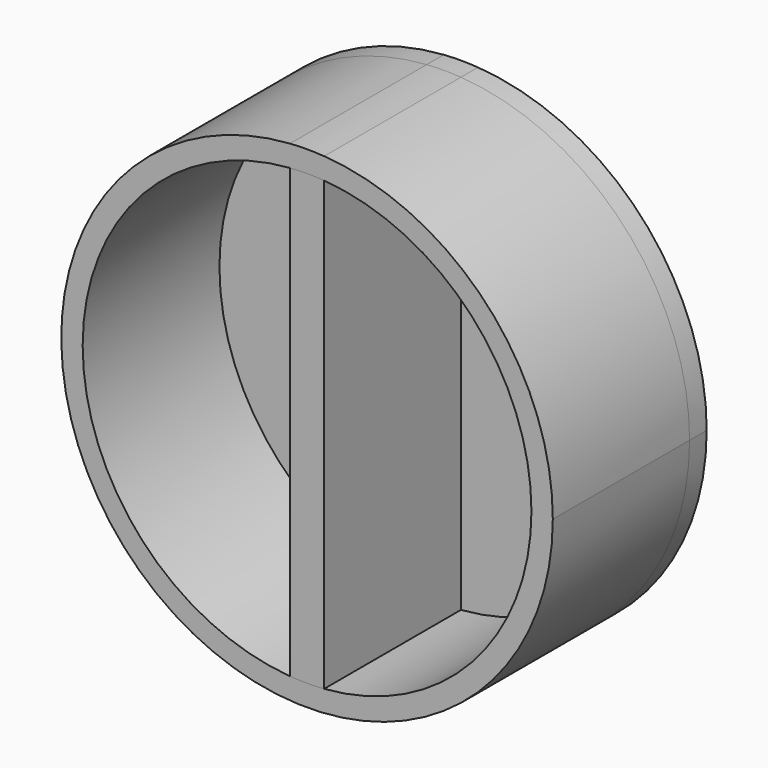
from build123d import *

# Parameters (mm, degrees)
F1_DEPTH = 6.35
F2_DEPTH = 50.8
F3_DEPTH = 50.8


with BuildPart() as f1:
    # F0 (on Front) → F1 (new body)
    with BuildSketch(Plane.XZ):
        with BuildLine():
            ThreePointArc((-5.08, 72.8480900573), (-49.8080496757, -53.4023296542), (73.025, 0))
            ThreePointArc((73.025, 0), (53.4023296542, 49.8080496757), (5.08, 72.8480900573))
            Line((5.08, 72.8480900573), (5.08, 66.4811945215))
            ThreePointArc((5.08, 66.4811945215), (48.909429689, 45.3147140838), (66.675, 0))
            ThreePointArc((66.675, 0), (48.909429689, -45.3147140838), (5.08, -66.4811945215))
            ThreePointArc((5.08, -66.4811945215), (0, -66.675), (-5.08, -66.4811945215))
            ThreePointArc((-5.08, -66.4811945215), (-66.675, 0), (-5.08, 66.4811945215))
            Line((-5.08, 66.4811945215), (-5.08, 72.8480900573))
        make_face()
        with BuildLine():
            Line((5.08, 66.4811945215), (5.08, 72.8480900573))
            ThreePointArc((5.08, 72.8480900573), (0, 73.025), (-5.08, 72.8480900573))
            Line((-5.08, 72.8480900573), (-5.08, 66.4811945215))
            ThreePointArc((-5.08, 66.4811945215), (0, 66.675), (5.08, 66.4811945215))
        make_face()
        with BuildLine():
            Line((5.08, -66.4811945215), (5.08, 66.4811945215))
            ThreePointArc((5.08, 66.4811945215), (0, 66.675), (-5.08, 66.4811945215))
            Line((-5.08, 66.4811945215), (-5.08, 0))
            Line((-5.08, 0), (-5.08, -66.4811945215))
            ThreePointArc((-5.08, -66.4811945215), (0, -66.675), (5.08, -66.4811945215))
        make_face()
        with BuildLine():
            ThreePointArc((66.675, 0), (48.909429689, 45.3147140838), (5.08, 66.4811945215))
            Line((5.08, 66.4811945215), (5.08, -66.4811945215))
            ThreePointArc((5.08, -66.4811945215), (48.909429689, -45.3147140838), (66.675, 0))
        make_face()
        with BuildLine():
            Line((-5.08, 0), (-5.08, 66.4811945215))
            ThreePointArc((-5.08, 66.4811945215), (-66.675, 0), (-5.08, -66.4811945215))
            Line((-5.08, -66.4811945215), (-5.08, 0))
        make_face()
    extrude(amount=-F1_DEPTH)


with BuildPart() as f2:
    # F0 (on Front) → F2 (new body)
    with BuildSketch(Plane.XZ):
        with BuildLine():
            ThreePointArc((-5.08, 72.8480900573), (-49.8080496757, -53.4023296542), (73.025, 0))
            ThreePointArc((73.025, 0), (53.4023296542, 49.8080496757), (5.08, 72.8480900573))
            Line((5.08, 72.8480900573), (5.08, 66.4811945215))
            ThreePointArc((5.08, 66.4811945215), (48.909429689, 45.3147140838), (66.675, 0))
            ThreePointArc((66.675, 0), (48.909429689, -45.3147140838), (5.08, -66.4811945215))
            ThreePointArc((5.08, -66.4811945215), (0, -66.675), (-5.08, -66.4811945215))
            ThreePointArc((-5.08, -66.4811945215), (-66.675, 0), (-5.08, 66.4811945215))
            Line((-5.08, 66.4811945215), (-5.08, 72.8480900573))
        make_face()
        with BuildLine():
            Line((5.08, 66.4811945215), (5.08, 72.8480900573))
            ThreePointArc((5.08, 72.8480900573), (0, 73.025), (-5.08, 72.8480900573))
            Line((-5.08, 72.8480900573), (-5.08, 66.4811945215))
            ThreePointArc((-5.08, 66.4811945215), (0, 66.675), (5.08, 66.4811945215))
        make_face()
    extrude(amount=F2_DEPTH)


with BuildPart() as f3:
    # F0 (on Front) → F3 (new body)
    with BuildSketch(Plane.XZ):
        with BuildLine():
            Line((5.08, -66.4811945215), (5.08, 66.4811945215))
            ThreePointArc((5.08, 66.4811945215), (0, 66.675), (-5.08, 66.4811945215))
            Line((-5.08, 66.4811945215), (-5.08, 0))
            Line((-5.08, 0), (-5.08, -66.4811945215))
            ThreePointArc((-5.08, -66.4811945215), (0, -66.675), (5.08, -66.4811945215))
        make_face()
    extrude(amount=F3_DEPTH)


solid = Compound([f1.part, f2.part, f3.part])
